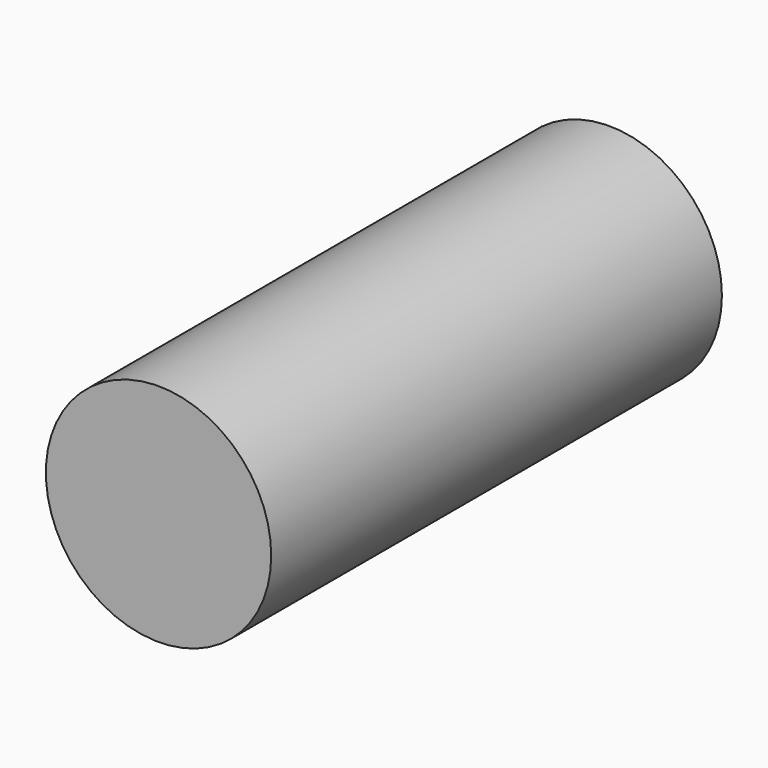
from build123d import *

# Parameters (mm, degrees)
F0_R     = 25.4
F1_DEPTH = 101.6
F3_DEPTH = 25.4


# Not quite as in the source:
# - the program builds the solid bodies; features that only make, move or delete a surface that nothing else refers to are left out


with BuildPart() as f1:
    # F0 (on Front) → F1 (new body)
    with BuildSketch(Plane.XZ):
        Circle(F0_R)
    extrude(amount=F1_DEPTH)

    # F3 (add): a face of the model
    f3_faces = [f1.faces().sort_by_distance(p)[0] for p in [
        (0, -101.6, 0),
    ]]
    extrude(f3_faces, amount=F3_DEPTH)


solid = f1.part
